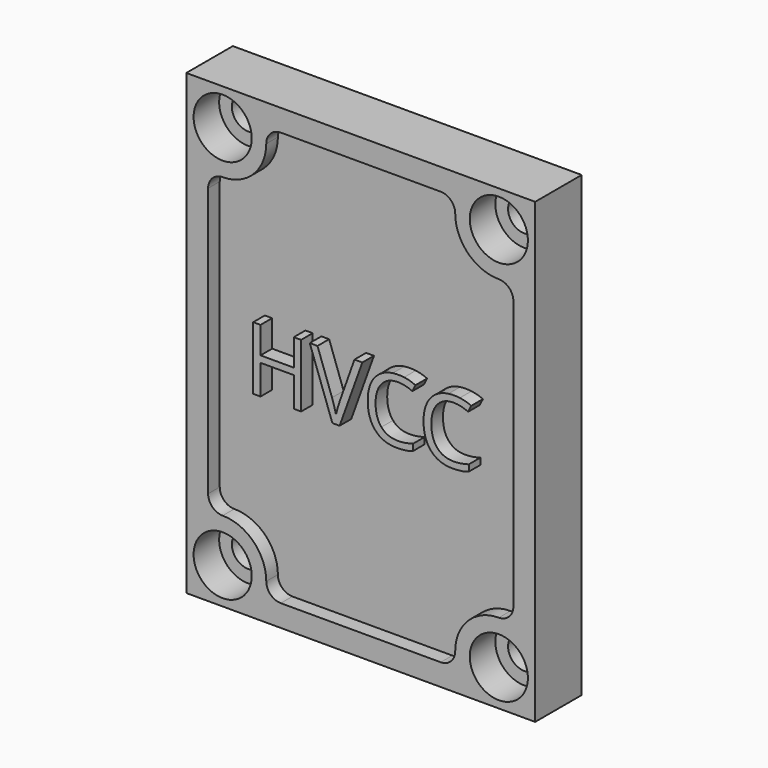
from build123d import *

# Parameters (mm, degrees)
F1_DEPTH  = 8
F2_R      = 2.25
F3_DEPTH  = 2
F5_DEPTH  = 2
F7_DEPTH  = 2
F2_R_2    = 4
F8_DEPTH  = 4.4
F9_DEPTH  = 8.001
F10_DEPTH = 8.001
F11_DEPTH = 4.4


# Not quite as in the source:
# - a feature names something its author has since deleted; it is built from what else it names


with BuildPart() as f1:
    # F0 (on Front) → F1 (new body)
    with BuildSketch(Plane.XZ):
        Polygon((24, 31.5), (0, 31.5), (-24, 31.5), (-24, -31.5), (0, -31.5), (24, -31.5), align=None)
    extrude(amount=F1_DEPTH)

    # F2 (on face) → F3 (cut)
    with BuildSketch(Plane.XZ.offset(8)):
        with Locations((-19, 26.5)):
            Circle(F2_R)
        with Locations((19, 26.5)):
            Circle(F2_R)
    extrude(amount=-F3_DEPTH, mode=Mode.SUBTRACT)

    # F4 (on face) → F5 (cut)
    with BuildSketch(Plane.XZ.offset(8)):
        with BuildLine():
            Line((-11, -28.5), (0, -28.5))
            Line((0, -28.5), (11, -28.5))
            ThreePointArc((11, -28.5), (12.4142135624, -27.9142135624), (13, -26.5))
            ThreePointArc((13, -26.5), (14.7573593129, -22.2573593129), (19, -20.5))
            ThreePointArc((19, -20.5), (20.4142135624, -19.9142135624), (21, -18.5))
            Line((21, -18.5), (21, 0))
            Line((21, 0), (21, 18.5))
            ThreePointArc((21, 18.5), (20.4142135624, 19.9142135624), (19, 20.5))
            ThreePointArc((19, 20.5), (14.7573593129, 22.2573593129), (13, 26.5))
            ThreePointArc((13, 26.5), (12.4142135624, 27.9142135624), (11, 28.5))
            Line((11, 28.5), (0, 28.5))
            Line((0, 28.5), (-11, 28.5))
            ThreePointArc((-11, 28.5), (-12.4142135624, 27.9142135624), (-13, 26.5))
            ThreePointArc((-13, 26.5), (-14.7573593129, 22.2573593129), (-19, 20.5))
            ThreePointArc((-19, 20.5), (-20.4142135624, 19.9142135624), (-21, 18.5))
            Line((-21, 18.5), (-21, 0))
            Line((-21, 0), (-21, -18.5))
            ThreePointArc((-21, -18.5), (-20.4142135624, -19.9142135624), (-19, -20.5))
            ThreePointArc((-19, -20.5), (-14.7573593129, -22.2573593129), (-13, -26.5))
            ThreePointArc((-13, -26.5), (-12.4142135624, -27.9142135624), (-11, -28.5))
        make_face()
    extrude(amount=-F5_DEPTH, mode=Mode.SUBTRACT)

    # F6 (on face) → F7 (join)
    with BuildSketch(Plane.XZ.offset(6)):
        Polygon((-9.214199551, -4.3776710518), (-8.2052831758, -4.3776710518), (-8.2052831758, 4.3035698491), (-9.214199551, 4.3035698491), (-9.214199551, 0.6099098991), (-13.7875737792, 0.6099098991), (-13.7875737792, 4.3035698491), (-14.7964901544, 4.3035698491), (-14.7964901544, -4.3776710518), (-13.7875737792, -4.3776710518), (-13.7875737792, -0.2926047491), (-9.214199551, -0.2926047491), align=None)
        with BuildLine():
            Line((-3.9055133884, -4.3776710518), (-2.9079971982, -4.3776710518))
            Line((-2.9079971982, -4.3776710518), (0.2194535618, 4.3035698491))
            Line((0.2194535618, 4.3035698491), (-0.8654640469, 4.3035698491))
            Line((-0.8654640469, 4.3035698491), (-2.8490962422, -1.2787207543))
            add(Edge.make_bspline(
                [(-3.4077053087, -3.1958518703), (-3.193001824, -2.234436266), (-2.8490962422, -1.2787207543)],
                knots=[0, 0, 0, 1, 1, 1], degree=2))
            add(Edge.make_bspline(
                [(-3.9530141594, -1.3129213094), (-3.6091085776, -2.281937037), (-3.4077053087, -3.1958518703)],
                knots=[0, 0, 0, 1, 1, 1], degree=2))
            Line((-3.9530141594, -1.3129213094), (-5.9480465397, 4.3035698491))
            Line((-5.9480465397, 4.3035698491), (-7.0177639018, 4.3035698491))
            Line((-7.0177639018, 4.3035698491), (-3.9055133884, -4.3776710518))
        make_face()
        with BuildLine():
            add(Edge.make_bspline(
                [(3.8245554648, -4.3776710518), (2.7125988005, -4.1239843021), (2.0045325346, -3.3326540906)],
                knots=[0.3205826669, 0.3205826669, 0.3205826669, 1, 1, 1], degree=2))
            Line((3.8245554648, -4.3776710518), (6.3867026136, -4.3776710518))
            add(Edge.make_bspline(
                [(7.1906667081, -4.1572674745), (6.8235762872, -4.2956026015), (6.3867026136, -4.3776710518)],
                knots=[0, 0, 0, 0.406741787, 0.406741787, 0.406741787], degree=2))
            Line((7.1906667081, -4.1572674745), (7.1906667081, -3.2737531346))
            add(Edge.make_bspline(
                [(5.1177330633, -3.6005584388), (6.0259478041, -3.6005584388), (7.1906667081, -3.2737531346)],
                knots=[0, 0, 0, 1, 1, 1], degree=2))
            add(Edge.make_bspline(
                [(2.8405461035, -2.6704933434), (3.639509071, -3.6005584388), (5.1177330633, -3.6005584388)],
                knots=[0, 0, 0, 1, 1, 1], degree=2))
            add(Edge.make_bspline(
                [(2.0415831359, -0.0380006168), (2.0415831359, -1.740428248), (2.8405461035, -2.6704933434)],
                knots=[0, 0, 0, 1, 1, 1], degree=2))
            add(Edge.make_bspline(
                [(2.8699965815, 2.5716917398), (2.0415831359, 1.6188262744), (2.0415831359, -0.0380006168)],
                knots=[0, 0, 0, 1, 1, 1], degree=2))
            add(Edge.make_bspline(
                [(5.1291332484, 3.5245572053), (3.698410027, 3.5245572053), (2.8699965815, 2.5716917398)],
                knots=[0, 0, 0, 1, 1, 1], degree=2))
            add(Edge.make_bspline(
                [(7.1013652587, 3.0628497116), (6.1152492535, 3.5245572053), (5.1291332484, 3.5245572053)],
                knots=[0, 0, 0, 1, 1, 1], degree=2))
            Line((7.1013652587, 3.0628497116), (7.5288721973, 3.9292637739))
            add(Edge.make_bspline(
                [(5.9680043466, 4.3776710518), (6.8286727205, 4.2702531102), (7.5288721973, 3.9292637739)],
                knots=[0.3150184776, 0.3150184776, 0.3150184776, 1, 1, 1], degree=2))
            Line((5.9680043466, 4.3776710518), (4.4013922849, 4.3776710518))
            add(Edge.make_bspline(
                [(2.9127472753, 3.8808129875), (3.5750775116, 4.2627988309), (4.4013922849, 4.3776710518)],
                knots=[0, 0, 0, 0.6992762354, 0.6992762354, 0.6992762354], degree=2))
            add(Edge.make_bspline(
                [(1.463973761, 2.3256377463), (1.9655819024, 3.3345541215), (2.9127472753, 3.8808129875)],
                knots=[0, 0, 0, 1, 1, 1], degree=2))
            add(Edge.make_bspline(
                [(0.9623656197, -0.0247004009), (0.9623656197, 1.316721371), (1.463973761, 2.3256377463)],
                knots=[0, 0, 0, 1, 1, 1], degree=2))
            add(Edge.make_bspline(
                [(2.0045325346, -3.3326540906), (0.9623656197, -2.1679351867), (0.9623656197, -0.0247004009)],
                knots=[0, 0, 0, 1, 1, 1], degree=2))
        make_face()
        with BuildLine():
            add(Edge.make_bspline(
                [(11.4968799904, -4.3776710518), (10.3849233261, -4.1239843021), (9.6768570602, -3.3326540906)],
                knots=[0.3205826669, 0.3205826669, 0.3205826669, 1, 1, 1], degree=2))
            Line((11.4968799904, -4.3776710518), (14.0590271393, -4.3776710518))
            add(Edge.make_bspline(
                [(14.8629912337, -4.1572674745), (14.4959008129, -4.2956026015), (14.0590271393, -4.3776710518)],
                knots=[0, 0, 0, 0.406741787, 0.406741787, 0.406741787], degree=2))
            Line((14.8629912337, -4.1572674745), (14.8629912337, -3.2737531346))
            add(Edge.make_bspline(
                [(12.790057589, -3.6005584388), (13.6982723297, -3.6005584388), (14.8629912337, -3.2737531346)],
                knots=[0, 0, 0, 1, 1, 1], degree=2))
            add(Edge.make_bspline(
                [(10.5128706291, -2.6704933434), (11.3118335967, -3.6005584388), (12.790057589, -3.6005584388)],
                knots=[0, 0, 0, 1, 1, 1], degree=2))
            add(Edge.make_bspline(
                [(9.7139076615, -0.0380006168), (9.7139076615, -1.740428248), (10.5128706291, -2.6704933434)],
                knots=[0, 0, 0, 1, 1, 1], degree=2))
            add(Edge.make_bspline(
                [(10.5423211071, 2.5716917398), (9.7139076615, 1.6188262744), (9.7139076615, -0.0380006168)],
                knots=[0, 0, 0, 1, 1, 1], degree=2))
            add(Edge.make_bspline(
                [(12.801457774, 3.5245572053), (11.3707345527, 3.5245572053), (10.5423211071, 2.5716917398)],
                knots=[0, 0, 0, 1, 1, 1], degree=2))
            add(Edge.make_bspline(
                [(14.7736897843, 3.0628497116), (13.7875737792, 3.5245572053), (12.801457774, 3.5245572053)],
                knots=[0, 0, 0, 1, 1, 1], degree=2))
            Line((14.7736897843, 3.0628497116), (15.201196723, 3.9292637739))
            add(Edge.make_bspline(
                [(13.6403288722, 4.3776710518), (14.5009972462, 4.2702531102), (15.201196723, 3.9292637739)],
                knots=[0.3150184776, 0.3150184776, 0.3150184776, 1, 1, 1], degree=2))
            Line((13.6403288722, 4.3776710518), (12.0737168105, 4.3776710518))
            add(Edge.make_bspline(
                [(10.585071801, 3.8808129875), (11.2474020372, 4.2627988309), (12.0737168105, 4.3776710518)],
                knots=[0, 0, 0, 0.6992762354, 0.6992762354, 0.6992762354], degree=2))
            add(Edge.make_bspline(
                [(9.1362982866, 2.3256377463), (9.637906428, 3.3345541215), (10.585071801, 3.8808129875)],
                knots=[0, 0, 0, 1, 1, 1], degree=2))
            add(Edge.make_bspline(
                [(8.6346901453, -0.0247004009), (8.6346901453, 1.316721371), (9.1362982866, 2.3256377463)],
                knots=[0, 0, 0, 1, 1, 1], degree=2))
            add(Edge.make_bspline(
                [(9.6768570602, -3.3326540906), (8.6346901453, -2.1679351867), (8.6346901453, -0.0247004009)],
                knots=[0, 0, 0, 1, 1, 1], degree=2))
        make_face()
        with BuildLine():
            Line((6.3867026136, -4.3776710518), (3.8245554648, -4.3776710518))
            add(Edge.make_bspline(
                [(4.9638305654, -4.4973729946), (4.3492315594, -4.4973729946), (3.8245554648, -4.3776710518)],
                knots=[0, 0, 0, 0.3205826669, 0.3205826669, 0.3205826669], degree=2))
            add(Edge.make_bspline(
                [(6.3867026136, -4.3776710518), (5.7494951686, -4.4973729946), (4.9638305654, -4.4973729946)],
                knots=[0.406741787, 0.406741787, 0.406741787, 1, 1, 1], degree=2))
        make_face()
        with BuildLine():
            Line((14.0590271393, -4.3776710518), (11.4968799904, -4.3776710518))
            add(Edge.make_bspline(
                [(12.6361550911, -4.4973729946), (12.0215560851, -4.4973729946), (11.4968799904, -4.3776710518)],
                knots=[0, 0, 0, 0.3205826669, 0.3205826669, 0.3205826669], degree=2))
            add(Edge.make_bspline(
                [(14.0590271393, -4.3776710518), (13.4218196942, -4.4973729946), (12.6361550911, -4.4973729946)],
                knots=[0.406741787, 0.406741787, 0.406741787, 1, 1, 1], degree=2))
        make_face()
        with BuildLine():
            add(Edge.make_bspline(
                [(4.4013922849, 4.3776710518), (4.7567489763, 4.4270718536), (5.1424334642, 4.4270718536)],
                knots=[0.6992762354, 0.6992762354, 0.6992762354, 1, 1, 1], degree=2))
            Line((4.4013922849, 4.3776710518), (5.9680043466, 4.3776710518))
            add(Edge.make_bspline(
                [(5.1424334642, 4.4270718536), (5.5721886465, 4.4270718536), (5.9680043466, 4.3776710518)],
                knots=[0, 0, 0, 0.3150184776, 0.3150184776, 0.3150184776], degree=2))
        make_face()
        with BuildLine():
            Line((12.0737168105, 4.3776710518), (13.6403288722, 4.3776710518))
            add(Edge.make_bspline(
                [(12.8147579899, 4.4270718536), (13.2445131721, 4.4270718536), (13.6403288722, 4.3776710518)],
                knots=[0, 0, 0, 0.3150184776, 0.3150184776, 0.3150184776], degree=2))
            add(Edge.make_bspline(
                [(12.0737168105, 4.3776710518), (12.4290735019, 4.4270718536), (12.8147579899, 4.4270718536)],
                knots=[0.6992762354, 0.6992762354, 0.6992762354, 1, 1, 1], degree=2))
        make_face()
    extrude(amount=F7_DEPTH)

    # F2 (on face) → F8 (cut)
    with BuildSketch(Plane.XZ.offset(8)):
        with Locations((-19, 26.5)):
            Circle(F2_R_2)
        with Locations((-19, 26.5)):
            Circle(F2_R, mode=Mode.SUBTRACT)
        with Locations((19, 26.5)):
            Circle(F2_R_2)
        with Locations((19, 26.5)):
            Circle(F2_R, mode=Mode.SUBTRACT)
    extrude(amount=-F8_DEPTH, mode=Mode.SUBTRACT)

    # F2 (on face) → F9 (cut, through all)
    with BuildSketch(Plane.XZ.offset(8)):
        with Locations((-19, 26.5)):
            Circle(F2_R)
        with Locations((19, 26.5)):
            Circle(F2_R)
    extrude(amount=-F9_DEPTH, mode=Mode.SUBTRACT)

    # F2 (on face) → F10 (cut, through all)
    with BuildSketch(Plane.XZ.offset(8)):
        with Locations((-19, -26.5)):
            Circle(F2_R)
        with Locations((19, -26.5)):
            Circle(F2_R)
    extrude(amount=-F10_DEPTH, mode=Mode.SUBTRACT)

    # F2 (on face) → F11 (cut)
    with BuildSketch(Plane.XZ.offset(8)):
        with Locations((-19, -26.5)):
            Circle(F2_R_2)
        with Locations((-19, -26.5)):
            Circle(F2_R, mode=Mode.SUBTRACT)
        with Locations((19, -26.5)):
            Circle(F2_R_2)
        with Locations((19, -26.5)):
            Circle(F2_R, mode=Mode.SUBTRACT)
    extrude(amount=-F11_DEPTH, mode=Mode.SUBTRACT)


solid = f1.part
